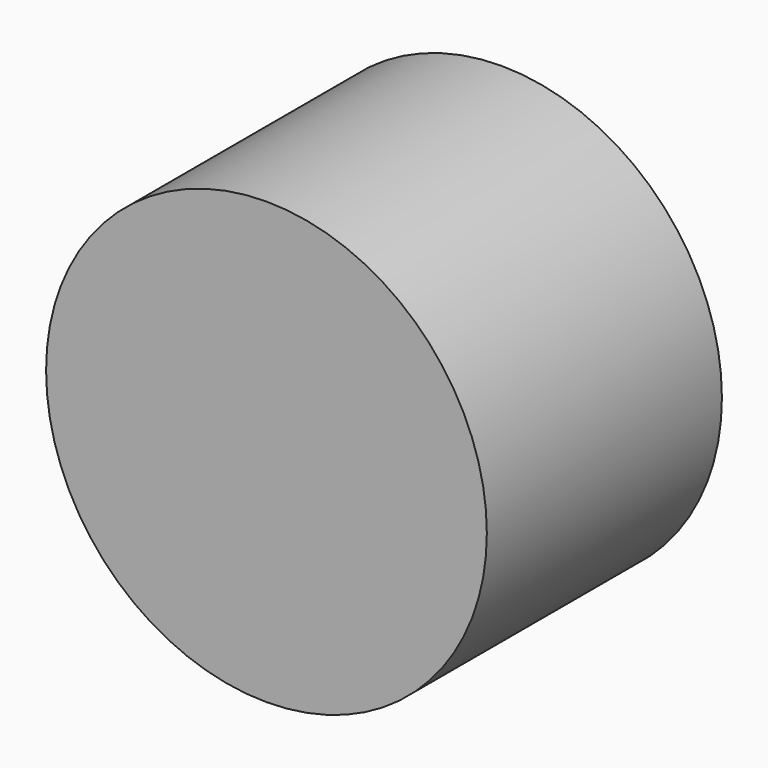
from build123d import *

# Parameters (mm, degrees)
F0_R     = 38.1
F1_DEPTH = 12.7
F2_DEPTH = 25.4
F3_DEPTH = 12.7


# Not quite as in the source:
# - the program builds the solid bodies; features that only make, move or delete a surface that nothing else refers to are left out


with BuildPart() as f1:
    # F0 (on Front) → F1 (new body)
    with BuildSketch(Plane.XZ):
        Circle(F0_R)
    extrude(amount=F1_DEPTH)

    # F2 (add): a face of the model
    f2_faces = [f1.faces().sort_by_distance(p)[0] for p in [
        (0, -12.7, 0),
    ]]
    extrude(f2_faces, amount=F2_DEPTH)

    # F3 (add): a face of the model
    f3_faces = [f1.faces().sort_by_distance(p)[0] for p in [
        (0, -38.1, 0),
    ]]
    extrude(f3_faces, amount=F3_DEPTH)


solid = f1.part
